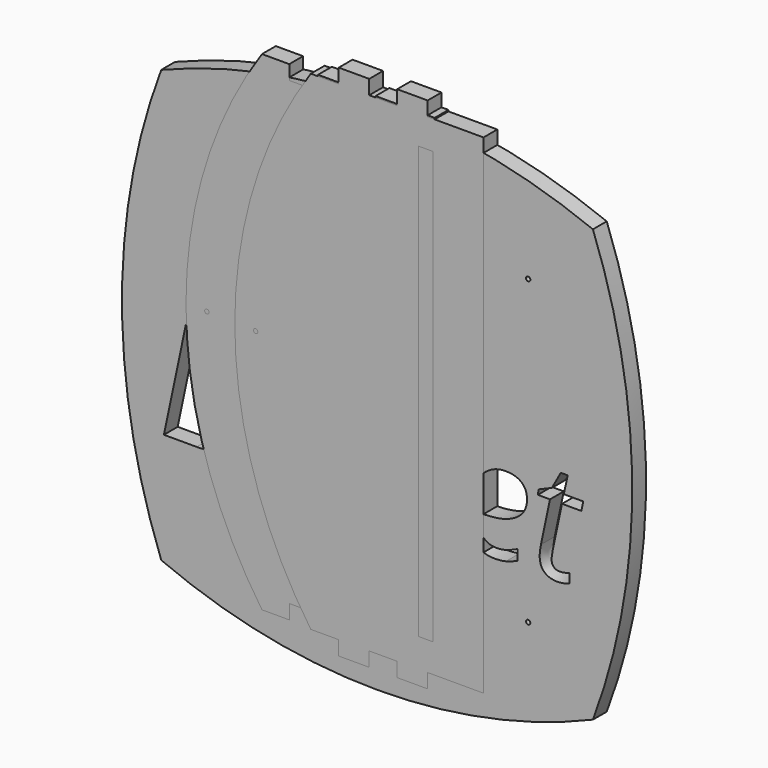
from build123d import *

# Parameters (mm, degrees)
F0_W     = 150
F0_H     = 150.000000298
F0_R     = 0.75
F3_DEPTH = 6
F1_R     = 0.75
F1_W     = 5
F1_H     = 150
F4_DEPTH = 6
F2_R     = 0.75
F2_W     = 5
F2_H     = 150
F5_DEPTH = 6


# Not quite as in the source:
# - ends of sketch curves that miss each other by under 0.0002 mm in the source are joined


with BuildPart() as f3:
    # F0 (on Front) → F3 (new body)
    with BuildSketch(Plane.XZ):
        with Locations((0, 1.49e-07)):
            Rectangle(F0_W, F0_H)
        with Locations((-52.5, -52.5)):
            Circle(F0_R, mode=Mode.SUBTRACT)
        with BuildLine():
            Line((-66.4784138573, -0.3075545752), (-57.236004571, -0.3075545752))
            add(Edge.make_bspline(
                [(-57.236004571, -0.3075545752), (-46.5898846592, -0.3075545752), (-46.5898846592, -8.5878700622)],
                knots=[0, 0, 0, 1, 1, 1], degree=2))
            add(Edge.make_bspline(
                [(-46.5898846592, -8.5878700622), (-46.5898846592, -12.0656025667), (-48.7309376637, -14.4550650358)],
                knots=[0, 0, 0, 1, 1, 1], degree=2))
            add(Edge.make_bspline(
                [(-48.7309376637, -14.4550650358), (-50.8719906682, -16.8445275048), (-54.7676819544, -17.562154847)],
                knots=[0, 0, 0, 1, 1, 1], degree=2))
            Line((-54.7676819544, -17.562154847), (-54.7676819544, -17.8066213043))
            add(Edge.make_bspline(
                [(-54.7676819544, -17.8066213043), (-51.9366026593, -18.5952227792), (-50.4185448201, -20.5312394002)],
                knots=[0, 0, 0, 1, 1, 1], degree=2))
            add(Edge.make_bspline(
                [(-50.4185448201, -20.5312394002), (-48.9004869808, -22.4672560212), (-48.9004869808, -25.1721590803)],
                knots=[0, 0, 0, 1, 1, 1], degree=2))
            add(Edge.make_bspline(
                [(-48.9004869808, -25.1721590803), (-48.9004869808, -30.4005868592), (-52.6463439868, -33.3696714123)],
                knots=[0, 0, 0, 1, 1, 1], degree=2))
            add(Edge.make_bspline(
                [(-52.6463439868, -33.3696714123), (-56.3922009928, -36.3387559655), (-62.6773547481, -36.3387559655)],
                knots=[0, 0, 0, 1, 1, 1], degree=2))
            Line((-62.6773547481, -36.3387559655), (-74.0884180906, -36.3387559655))
            Line((-74.0884180906, -36.3387559655), (-66.4784138573, -0.3075545752))
        make_face(mode=Mode.SUBTRACT)
        with BuildLine():
            add(Edge.make_bspline(
                [(-37.0280917755, -11.3243171802), (-33.9486030158, -8.8323365194), (-30.2737201426, -8.8323365194)],
                knots=[0, 0, 0, 1, 1, 1], degree=2))
            add(Edge.make_bspline(
                [(-30.2737201426, -8.8323365194), (-28.0104339095, -8.8323365194), (-26.2360805909, -10.0546688056)],
                knots=[0, 0, 0, 1, 1, 1], degree=2))
            add(Edge.make_bspline(
                [(-26.2360805909, -10.0546688056), (-24.4617272722, -11.2770010917), (-23.4759754285, -13.5639453691)],
                knots=[0, 0, 0, 1, 1, 1], degree=2))
            Line((-23.4759754285, -13.5639453691), (-23.1999649123, -13.5639453691))
            Line((-23.1999649123, -13.5639453691), (-21.5517878297, -9.3291554486))
            Line((-21.5517878297, -9.3291554486), (-18.4210399741, -9.3291554486))
            Line((-18.4210399741, -9.3291554486), (-24.1620587117, -36.3387559655))
            Line((-24.1620587117, -36.3387559655), (-27.4426408475, -36.3387559655))
            Line((-27.4426408475, -36.3387559655), (-26.7959876381, -31.1891883341))
            Line((-26.7959876381, -31.1891883341), (-26.9931380068, -31.1891883341))
            add(Edge.make_bspline(
                [(-26.9931380068, -31.1891883341), (-31.4093062665, -36.8355748947), (-36.2907493964, -36.8355748947)],
                knots=[0, 0, 0, 1, 1, 1], degree=2))
            add(Edge.make_bspline(
                [(-36.2907493964, -36.8355748947), (-39.7132797977, -36.8355748947), (-41.6611254408, -34.3948533298)],
                knots=[0, 0, 0, 1, 1, 1], degree=2))
            add(Edge.make_bspline(
                [(-41.6611254408, -34.3948533298), (-43.6089710839, -31.9541317648), (-43.6089710839, -27.7114558296)],
                knots=[0, 0, 0, 1, 1, 1], degree=2))
            add(Edge.make_bspline(
                [(-43.6089710839, -27.7114558296), (-43.6089710839, -22.5855462424), (-41.8582758095, -18.2009220417)],
                knots=[0, 0, 0, 1, 1, 1], degree=2))
            add(Edge.make_bspline(
                [(-41.8582758095, -18.2009220417), (-40.1075805352, -13.8162978411), (-37.0280917755, -11.3243171802)],
                knots=[0, 0, 0, 1, 1, 1], degree=2))
        make_face(mode=Mode.SUBTRACT)
        with BuildLine():
            add(Edge.make_bspline(
                [(0.0401205543, -25.9252734888), (0.6079136163, -27.1436627676), (0.6079136163, -28.673549629)],
                knots=[0, 0, 0, 1, 1, 1], degree=2))
            add(Edge.make_bspline(
                [(0.6079136163, -28.673549629), (0.6079136163, -32.5219248268), (-2.1167044796, -34.6787498607)],
                knots=[0, 0, 0, 1, 1, 1], degree=2))
            add(Edge.make_bspline(
                [(-2.1167044796, -34.6787498607), (-4.8413225756, -36.8355748947), (-9.7937398382, -36.8355748947)],
                knots=[0, 0, 0, 1, 1, 1], degree=2))
            add(Edge.make_bspline(
                [(-9.7937398382, -36.8355748947), (-13.9575556259, -36.8355748947), (-17.3091118945, -35.1321957088)],
                knots=[0, 0, 0, 1, 1, 1], degree=2))
            Line((-17.3091118945, -35.1321957088), (-17.3091118945, -31.2365044226))
            add(Edge.make_bspline(
                [(-17.3091118945, -31.2365044226), (-15.5820746643, -32.2695723548), (-13.5869129327, -32.8373654167)],
                knots=[0, 0, 0, 1, 1, 1], degree=2))
            add(Edge.make_bspline(
                [(-13.5869129327, -32.8373654167), (-11.5917512011, -33.4051584787), (-9.8883720152, -33.4051584787)],
                knots=[0, 0, 0, 1, 1, 1], degree=2))
            add(Edge.make_bspline(
                [(-9.8883720152, -33.4051584787), (-6.7891682187, -33.4051584787), (-5.2119652688, -32.1749401778)],
                knots=[0, 0, 0, 1, 1, 1], degree=2))
            add(Edge.make_bspline(
                [(-5.2119652688, -32.1749401778), (-3.6347623189, -30.9447218769), (-3.6347623189, -29.020534278)],
                knots=[0, 0, 0, 1, 1, 1], degree=2))
            add(Edge.make_bspline(
                [(-3.6347623189, -29.020534278), (-3.6347623189, -27.6168236526), (-4.4943379266, -26.6547298532)],
                knots=[0, 0, 0, 1, 1, 1], degree=2))
            add(Edge.make_bspline(
                [(-4.4943379266, -26.6547298532), (-5.3539135343, -25.6926360537), (-8.2165368883, -24.0129149121)],
                knots=[0, 0, 0, 1, 1, 1], degree=2))
            add(Edge.make_bspline(
                [(-8.2165368883, -24.0129149121), (-11.4182588766, -22.2149035492), (-12.7509953693, -20.4918093265)],
                knots=[0, 0, 0, 1, 1, 1], degree=2))
            add(Edge.make_bspline(
                [(-12.7509953693, -20.4918093265), (-14.0837318619, -18.7687151037), (-14.0837318619, -16.4029106789)],
                knots=[0, 0, 0, 1, 1, 1], degree=2))
            add(Edge.make_bspline(
                [(-14.0837318619, -16.4029106789), (-14.0837318619, -13.0040383219), (-11.5917512011, -10.9181874206)],
                knots=[0, 0, 0, 1, 1, 1], degree=2))
            add(Edge.make_bspline(
                [(-11.5917512011, -10.9181874206), (-9.0997705403, -8.8323365194), (-5.0384729443, -8.8323365194)],
                knots=[0, 0, 0, 1, 1, 1], degree=2))
            add(Edge.make_bspline(
                [(-5.0384729443, -8.8323365194), (-0.8194550534, -8.8323365194), (3.0998942771, -10.6618919413)],
                knots=[0, 0, 0, 1, 1, 1], degree=2))
            Line((3.0998942771, -10.6618919413), (1.7671577845, -14.037106254))
            Line((1.7671577845, -14.037106254), (0.3871052033, -13.4219971036))
            add(Edge.make_bspline(
                [(0.3871052033, -13.4219971036), (-2.1048754575, -12.3573851124), (-5.0384729443, -12.3573851124)],
                knots=[0, 0, 0, 1, 1, 1], degree=2))
            add(Edge.make_bspline(
                [(-5.0384729443, -12.3573851124), (-7.3254172217, -12.3573851124), (-8.6344956701, -13.4298831183)],
                knots=[0, 0, 0, 1, 1, 1], degree=2))
            add(Edge.make_bspline(
                [(-8.6344956701, -13.4298831183), (-9.9435741185, -14.5023811243), (-9.9435741185, -16.2057603101)],
                knots=[0, 0, 0, 1, 1, 1], degree=2))
            add(Edge.make_bspline(
                [(-9.9435741185, -16.2057603101), (-9.9435741185, -17.5858128913), (-9.0682264813, -18.571564735)],
                knots=[0, 0, 0, 1, 1, 1], degree=2))
            add(Edge.make_bspline(
                [(-9.0682264813, -18.571564735), (-8.1928788441, -19.5573165787), (-5.456431726, -21.1108614843)],
                knots=[0, 0, 0, 1, 1, 1], degree=2))
            add(Edge.make_bspline(
                [(-5.456431726, -21.1108614843), (-2.814616785, -22.5855462424), (-1.6711446463, -23.6462152262)],
                knots=[0, 0, 0, 1, 1, 1], degree=2))
            add(Edge.make_bspline(
                [(-1.6711446463, -23.6462152262), (-0.5276725076, -24.7068842101), (0.0401205543, -25.9252734888)],
                knots=[0, 0, 0, 1, 1, 1], degree=2))
        make_face(mode=Mode.SUBTRACT)
        with Locations((52.5, -52.5)):
            Circle(F0_R, mode=Mode.SUBTRACT)
        with BuildLine():
            Line((12.1451531948, -22.5618881982), (12.2397853718, -22.5618881982))
            Line((12.2397853718, -22.5618881982), (25.2043936199, -9.3291554486))
            Line((25.2043936199, -9.3291554486), (30.1568108825, -9.3291554486))
            Line((30.1568108825, -9.3291554486), (18.6037992746, -20.8348509681))
            Line((18.6037992746, -20.8348509681), (25.8668188588, -36.3387559655))
            Line((25.8668188588, -36.3387559655), (21.2613862451, -36.3387559655))
            Line((21.2613862451, -36.3387559655), (15.473051419, -23.4214638059))
            Line((15.473051419, -23.4214638059), (11.727194413, -26.4575794844))
            Line((11.727194413, -26.4575794844), (9.7004886224, -36.3387559655))
            Line((9.7004886224, -36.3387559655), (5.5130147905, -36.3387559655))
            Line((5.5130147905, -36.3387559655), (13.6434959972, 2.0109337611))
            Line((13.6434959972, 2.0109337611), (17.8388558439, 2.0109337611))
            add(Edge.make_bspline(
                [(17.8388558439, 2.0109337611), (16.0645025252, -6.2693817258), (14.6568488925, -12.82660299)],
                knots=[0, 0, 0, 1, 1, 1], degree=2))
            add(Edge.make_bspline(
                [(14.6568488925, -12.82660299), (13.2491952597, -19.3838242542), (12.1451531948, -22.5618881982)],
                knots=[0, 0, 0, 1, 1, 1], degree=2))
        make_face(mode=Mode.SUBTRACT)
        with BuildLine():
            add(Edge.make_bspline(
                [(44.7695962133, -36.4018440835), (42.9952428946, -36.8355748947), (40.8581328975, -36.8355748947)],
                knots=[0, 0, 0, 1, 1, 1], degree=2))
            add(Edge.make_bspline(
                [(40.8581328975, -36.8355748947), (36.3236744166, -36.8355748947), (33.7331185714, -34.1464438652)],
                knots=[0, 0, 0, 1, 1, 1], degree=2))
            add(Edge.make_bspline(
                [(33.7331185714, -34.1464438652), (31.1425627262, -31.4573128356), (31.1425627262, -26.7020459417)],
                knots=[0, 0, 0, 1, 1, 1], degree=2))
            add(Edge.make_bspline(
                [(31.1425627262, -26.7020459417), (31.1425627262, -22.0729552837), (32.9800041628, -17.8184503264)],
                knots=[0, 0, 0, 1, 1, 1], degree=2))
            add(Edge.make_bspline(
                [(32.9800041628, -17.8184503264), (34.8174455994, -13.5639453691), (37.8496182706, -11.1981409442)],
                knots=[0, 0, 0, 1, 1, 1], degree=2))
            add(Edge.make_bspline(
                [(37.8496182706, -11.1981409442), (40.8817909418, -8.8323365194), (44.525129756, -8.8323365194)],
                knots=[0, 0, 0, 1, 1, 1], degree=2))
            add(Edge.make_bspline(
                [(44.525129756, -8.8323365194), (48.2946448063, -8.8323365194), (50.1951743609, -10.4726275873)],
                knots=[0, 0, 0, 1, 1, 1], degree=2))
            add(Edge.make_bspline(
                [(50.1951743609, -10.4726275873), (52.0957039155, -12.1129186552), (52.0957039155, -15.046516142)],
                knots=[0, 0, 0, 1, 1, 1], degree=2))
            add(Edge.make_bspline(
                [(52.0957039155, -15.046516142), (52.0957039155, -19.4784564312), (48.0028622605, -22.0059241584)],
                knots=[0, 0, 0, 1, 1, 1], degree=2))
            add(Edge.make_bspline(
                [(48.0028622605, -22.0059241584), (43.9100206056, -24.5333918856), (36.2921303576, -24.5333918856)],
                knots=[0, 0, 0, 1, 1, 1], degree=2))
            Line((36.2921303576, -24.5333918856), (35.4798708384, -24.5333918856))
            Line((35.4798708384, -24.5333918856), (35.3852386614, -26.5048955729))
            add(Edge.make_bspline(
                [(35.3852386614, -26.5048955729), (35.3852386614, -29.7302756055), (36.8993534933, -31.5440589978)],
                knots=[0, 0, 0, 1, 1, 1], degree=2))
            add(Edge.make_bspline(
                [(36.8993534933, -31.5440589978), (38.4134683252, -33.3578423902), (41.5915322692, -33.3578423902)],
                knots=[0, 0, 0, 1, 1, 1], degree=2))
            add(Edge.make_bspline(
                [(41.5915322692, -33.3578423902), (43.1450771749, -33.3578423902), (44.7853682428, -32.9122825569)],
                knots=[0, 0, 0, 1, 1, 1], degree=2))
            add(Edge.make_bspline(
                [(44.7853682428, -32.9122825569), (46.4256593107, -32.4667227235), (48.8624378682, -31.2838205111)],
                knots=[0, 0, 0, 1, 1, 1], degree=2))
            Line((48.8624378682, -31.2838205111), (48.8624378682, -34.8877292516))
            add(Edge.make_bspline(
                [(48.8624378682, -34.8877292516), (46.5439495319, -35.9681132723), (44.7695962133, -36.4018440835)],
                knots=[0, 0, 0, 1, 1, 1], degree=2))
        make_face(mode=Mode.SUBTRACT)
        with BuildLine():
            add(Edge.make_bspline(
                [(61.3578282387, -32.7151321881), (62.0715125736, -33.4524745672), (63.349046963, -33.4524745672)],
                knots=[0, 0, 0, 1, 1, 1], degree=2))
            add(Edge.make_bspline(
                [(63.349046963, -33.4524745672), (64.7054414999, -33.4524745672), (66.8977536002, -32.8137073725)],
                knots=[0, 0, 0, 1, 1, 1], degree=2))
            Line((66.8977536002, -32.8137073725), (66.8977536002, -35.9917713165))
            add(Edge.make_bspline(
                [(66.8977536002, -35.9917713165), (66.0618360368, -36.3387559655), (64.8316177359, -36.5871654301)],
                knots=[0, 0, 0, 1, 1, 1], degree=2))
            add(Edge.make_bspline(
                [(64.8316177359, -36.5871654301), (63.601399435, -36.8355748947), (62.8601140485, -36.8355748947)],
                knots=[0, 0, 0, 1, 1, 1], degree=2))
            add(Edge.make_bspline(
                [(62.8601140485, -36.8355748947), (59.7766822815, -36.8355748947), (58.140334221, -35.3687761513)],
                knots=[0, 0, 0, 1, 1, 1], degree=2))
            add(Edge.make_bspline(
                [(58.140334221, -35.3687761513), (56.5039861605, -33.9019774079), (56.5039861605, -30.9920379654)],
                knots=[0, 0, 0, 1, 1, 1], degree=2))
            add(Edge.make_bspline(
                [(56.5039861605, -30.9920379654), (56.5039861605, -29.367518927), (56.9456029864, -27.2934970479)],
                knots=[0, 0, 0, 1, 1, 1], degree=2))
            Line((56.9456029864, -27.2934970479), (60.076350842, -12.4599033041))
            Line((60.076350842, -12.4599033041), (55.8336749068, -12.4599033041))
            Line((55.8336749068, -12.4599033041), (56.1806595557, -10.6618919413))
            Line((56.1806595557, -10.6618919413), (60.7387760809, -8.7377043424))
            Line((60.7387760809, -8.7377043424), (63.822207848, -3.114975826))
            Line((63.822207848, -3.114975826), (66.2353283613, -3.114975826))
            Line((66.2353283613, -3.114975826), (64.8789338244, -9.3291554486))
            Line((64.8789338244, -9.3291554486), (71.6293624499, -9.3291554486))
            Line((71.6293624499, -9.3291554486), (70.9905952552, -12.4599033041))
            Line((70.9905952552, -12.4599033041), (64.2638246739, -12.4599033041))
            Line((64.2638246739, -12.4599033041), (61.0857607299, -27.3408131364))
            add(Edge.make_bspline(
                [(61.0857607299, -27.3408131364), (60.6441439039, -29.4858091482), (60.6441439039, -30.5977372279)],
                knots=[0, 0, 0, 1, 1, 1], degree=2))
            add(Edge.make_bspline(
                [(60.6441439039, -30.5977372279), (60.6441439039, -31.9777898091), (61.3578282387, -32.7151321881)],
                knots=[0, 0, 0, 1, 1, 1], degree=2))
        make_face(mode=Mode.SUBTRACT)
        Polygon((-9.8206784108, 13.3505715057), (-23.3275989091, 13.3505715057), (-17.6531634364, 40.217406402), (-14.5248736214, 40.217406402), (-19.5995242048, 16.1789688761), (-9.2150132775, 16.1789688761), align=None, mode=Mode.SUBTRACT)
        Polygon((1.4047074104, 33.4904072509), (-2.8996312073, 13.3505715057), (-5.9867593142, 13.3505715057), (-1.6824206965, 33.4904072509), align=None, mode=Mode.SUBTRACT)
        with Locations((-52.5, 52.5)):
            Circle(F0_R, mode=Mode.SUBTRACT)
        with BuildLine():
            add(Edge.make_bspline(
                [(4.4918355173, 5.906182585), (3.004133782, 4.3067562134), (0.5755930045, 4.3067562134)],
                knots=[0, 0, 0, 1, 1, 1], degree=2))
            add(Edge.make_bspline(
                [(0.5755930045, 4.3067562134), (-0.6945397023, 4.3067562134), (-1.7235824046, 4.6948523183)],
                knots=[0, 0, 0, 1, 1, 1], degree=2))
            Line((-1.7235824046, 4.6948523183), (-1.7235824046, 7.2880399281))
            add(Edge.make_bspline(
                [(-1.7235824046, 7.2880399281), (-0.547533602, 6.8823030912), (0.334503, 6.8823030912)],
                knots=[0, 0, 0, 1, 1, 1], degree=2))
            add(Edge.make_bspline(
                [(0.334503, 6.8823030912), (1.7340010751, 6.8823030912), (2.4866723088, 8.0201303078)],
                knots=[0, 0, 0, 1, 1, 1], degree=2))
            add(Edge.make_bspline(
                [(2.4866723088, 8.0201303078), (3.2393435425, 9.1579575243), (3.6980025755, 11.2748453691)],
                knots=[0, 0, 0, 1, 1, 1], degree=2))
            Line((3.6980025755, 11.2748453691), (7.8729758249, 31.1559503777))
            Line((7.8729758249, 31.1559503777), (4.3271886849, 31.1559503777))
            Line((4.3271886849, 31.1559503777), (4.5623984455, 32.3908016204))
            Line((4.5623984455, 32.3908016204), (8.34927559, 33.6021318872))
            Line((8.34927559, 33.6021318872), (8.7726531589, 35.4367680193))
            add(Edge.make_bspline(
                [(8.7726531589, 35.4367680193), (9.6194082968, 39.1119205275), (11.1159303982, 40.6290234829)],
                knots=[0, 0, 0, 1, 1, 1], degree=2))
            add(Edge.make_bspline(
                [(11.1159303982, 40.6290234829), (12.6124524995, 42.1461264383), (15.5525745061, 42.1461264383)],
                knots=[0, 0, 0, 1, 1, 1], degree=2))
            add(Edge.make_bspline(
                [(15.5525745061, 42.1461264383), (16.2876050078, 42.1461264383), (17.3519291742, 41.9344376539)],
                knots=[0, 0, 0, 1, 1, 1], degree=2))
            add(Edge.make_bspline(
                [(17.3519291742, 41.9344376539), (18.4162533405, 41.7227488694), (19.0042777419, 41.4640181328)],
                knots=[0, 0, 0, 1, 1, 1], degree=2))
            Line((19.0042777419, 41.4640181328), (18.2163250441, 39.0942797955))
            add(Edge.make_bspline(
                [(18.2163250441, 39.0942797955), (16.822707213, 39.6293820007), (15.6995806065, 39.6293820007)],
                knots=[0, 0, 0, 1, 1, 1], degree=2))
            add(Edge.make_bspline(
                [(15.6995806065, 39.6293820007), (14.1001542349, 39.6293820007), (13.2445787309, 38.7385250327)],
                knots=[0, 0, 0, 1, 1, 1], degree=2))
            add(Edge.make_bspline(
                [(13.2445787309, 38.7385250327), (12.389003227, 37.8476680647), (11.8597812658, 35.4779297274)],
                knots=[0, 0, 0, 1, 1, 1], degree=2))
            Line((11.8597812658, 35.4779297274), (11.4011222328, 33.4904072509))
            Line((11.4011222328, 33.4904072509), (15.7701435346, 33.4904072509))
            Line((15.7701435346, 33.4904072509), (15.3114845016, 31.1559503777))
            Line((15.3114845016, 31.1559503777), (10.9601039318, 31.1559503777))
            Line((10.9601039318, 31.1559503777), (6.6969270223, 10.9808331684))
            add(Edge.make_bspline(
                [(6.6969270223, 10.9808331684), (5.9795372526, 7.5056089566), (4.4918355173, 5.906182585)],
                knots=[0, 0, 0, 1, 1, 1], degree=2))
        make_face(mode=Mode.SUBTRACT)
        with BuildLine():
            add(Edge.make_bspline(
                [(20.0362605662, 16.0525436298), (20.5684226494, 15.5027408146), (21.5210221795, 15.5027408146)],
                knots=[0, 0, 0, 1, 1, 1], degree=2))
            add(Edge.make_bspline(
                [(21.5210221795, 15.5027408146), (22.5324241498, 15.5027408146), (24.1671319855, 15.9790405796)],
                knots=[0, 0, 0, 1, 1, 1], degree=2))
            Line((24.1671319855, 15.9790405796), (24.1671319855, 13.6093022423))
            add(Edge.make_bspline(
                [(24.1671319855, 13.6093022423), (23.5438261201, 13.3505715057), (22.626508054, 13.1653438193)],
                knots=[0, 0, 0, 1, 1, 1], degree=2))
            add(Edge.make_bspline(
                [(22.626508054, 13.1653438193), (21.7091899879, 12.9801161329), (21.1564470507, 12.9801161329)],
                knots=[0, 0, 0, 1, 1, 1], degree=2))
            add(Edge.make_bspline(
                [(21.1564470507, 12.9801161329), (18.8572716415, 12.9801161329), (17.6371210088, 14.0738415193)],
                knots=[0, 0, 0, 1, 1, 1], degree=2))
            add(Edge.make_bspline(
                [(17.6371210088, 14.0738415193), (16.4169703761, 15.1675669058), (16.4169703761, 17.3373769467)],
                knots=[0, 0, 0, 1, 1, 1], degree=2))
            add(Edge.make_bspline(
                [(16.4169703761, 17.3373769467), (16.4169703761, 18.5487072134), (16.7462640408, 20.0952113889)],
                knots=[0, 0, 0, 1, 1, 1], degree=2))
            Line((16.7462640408, 20.0952113889), (19.080720914, 31.1559503777))
            Line((19.080720914, 31.1559503777), (15.9171496349, 31.1559503777))
            Line((15.9171496349, 31.1559503777), (16.1758803715, 32.4966460127))
            Line((16.1758803715, 32.4966460127), (19.5746614111, 33.9314255519))
            Line((19.5746614111, 33.9314255519), (21.8738368203, 38.1240395333))
            Line((21.8738368203, 38.1240395333), (23.6731914883, 38.1240395333))
            Line((23.6731914883, 38.1240395333), (22.6617895181, 33.4904072509))
            Line((22.6617895181, 33.4904072509), (27.6952783934, 33.4904072509))
            Line((27.6952783934, 33.4904072509), (27.2189786283, 31.1559503777))
            Line((27.2189786283, 31.1559503777), (22.203130485, 31.1559503777))
            Line((22.203130485, 31.1559503777), (19.8333921477, 20.0599299248))
            add(Edge.make_bspline(
                [(19.8333921477, 20.0599299248), (19.504098483, 18.4605035532), (19.504098483, 17.6313891473)],
                knots=[0, 0, 0, 1, 1, 1], degree=2))
            add(Edge.make_bspline(
                [(19.504098483, 17.6313891473), (19.504098483, 16.602346445), (20.0362605662, 16.0525436298)],
                knots=[0, 0, 0, 1, 1, 1], degree=2))
        make_face(mode=Mode.SUBTRACT)
        with BuildLine():
            add(Edge.make_bspline(
                [(-0.3417250615, 37.3566676896), (-0.8180248266, 37.8065063566), (-0.8180248266, 38.6356207625)],
                knots=[0, 0, 0, 1, 1, 1], degree=2))
            add(Edge.make_bspline(
                [(-0.8180248266, 38.6356207625), (-0.8180248266, 39.6646634648), (-0.2300004253, 40.3173705502)],
                knots=[0, 0, 0, 1, 1, 1], degree=2))
            add(Edge.make_bspline(
                [(-0.2300004253, 40.3173705502), (0.358023976, 40.9700776357), (1.2929827741, 40.9700776357)],
                knots=[0, 0, 0, 1, 1, 1], degree=2))
            add(Edge.make_bspline(
                [(1.2929827741, 40.9700776357), (2.9100498778, 40.9700776357), (2.9100498778, 39.317729068)],
                knots=[0, 0, 0, 1, 1, 1], degree=2))
            add(Edge.make_bspline(
                [(2.9100498778, 39.317729068), (2.9100498778, 38.3063270977), (2.2955643784, 37.6065780601)],
                knots=[0, 0, 0, 1, 1, 1], degree=2))
            add(Edge.make_bspline(
                [(2.2955643784, 37.6065780601), (1.681078879, 36.9068290226), (0.8696052052, 36.9068290226)],
                knots=[0, 0, 0, 1, 1, 1], degree=2))
            add(Edge.make_bspline(
                [(0.8696052052, 36.9068290226), (0.1345747035, 36.9068290226), (-0.3417250615, 37.3566676896)],
                knots=[0, 0, 0, 1, 1, 1], degree=2))
        make_face(mode=Mode.SUBTRACT)
        with Locations((52.5, 52.5)):
            Circle(F0_R, mode=Mode.SUBTRACT)
        with BuildLine():
            ThreePointArc((75, 75.000000298), (-2.88e-08, 89.4985285534), (-75, 75))
            Line((-75, 75), (75, 75.000000298))
        make_face()
        with BuildLine():
            Line((-75, -75), (-75, 75))
            ThreePointArc((-75, 75), (-88.6491712085, -3.0074e-06), (-75, -75))
        make_face()
        with BuildLine():
            Line((75, -75), (-75, -75))
            ThreePointArc((-75, -75), (0, -90.2725273781), (75, -75))
        make_face()
        with BuildLine():
            ThreePointArc((74.9999931729, -74.9999970198), (88.6491640834, 3.0074e-06), (74.9999928749, 75.0000029802))
            Line((74.9999928749, 75.0000029802), (74.9999931729, -74.9999970198))
        make_face()
    extrude(amount=F3_DEPTH)


with BuildPart() as f4:
    # F1 (on Front) → F4 (new body)
    with BuildSketch(Plane.XZ):
        with BuildLine():
            Line((20.0000001626, -78.7899424732), (19.9999998374, 91.2100575268))
            Line((19.9999998374, 91.2100575268), (-0.5218474052, 91.2100575268))
            Line((-0.5218474052, 91.2100575268), (-0.5218474052, 88.210016489))
            Line((-0.5218474052, 88.210016489), (-0.5218474052, 86.2100575268))
            Line((-0.5218474052, 86.2100575268), (-10.5218474052, 86.2100575268))
            Line((-10.5218474052, 86.2100575268), (-10.5218474052, 88.210016489))
            Line((-10.5218474052, 88.210016489), (-10.5218474052, 91.2100575268))
            Line((-10.5218474052, 91.2100575268), (-20.5218474052, 91.2100575268))
            Line((-20.5218474052, 91.2100575268), (-20.5218474052, 88.210016489))
            Line((-20.5218474052, 88.210016489), (-20.5218474052, 86.2100575268))
            Line((-20.5218474052, 86.2100575268), (-30.5218474052, 86.2100575268))
            Line((-30.5218474052, 86.2100575268), (-30.5218474052, 88.210016489))
            Line((-30.5218474052, 88.210016489), (-30.5218474052, 91.2100575268))
            Line((-30.5218474052, 91.2100575268), (-40.0000001626, 91.2100575268))
            ThreePointArc((-40.0000001626, 91.2100575268), (-66.4079290569, 6.2100574763), (-39.9999998374, -78.7899424732))
            Line((-39.9999998374, -78.7899424732), (-30.5218463486, -78.7899435368))
            Line((-30.5218463486, -78.7899435368), (-30.5218463486, -75.7881775498))
            Line((-30.5218463486, -75.7881775498), (-30.5218463486, -73.7881775498))
            Line((-30.5218463486, -73.7881775498), (-20.5218463486, -73.7881775498))
            Line((-20.5218463486, -73.7881775498), (-20.5218463486, -75.7881775498))
            Line((-20.5218463486, -75.7881775498), (-20.5218463486, -78.7899435368))
            Line((-20.5218463486, -78.7899435368), (-10.5218463486, -78.7899435368))
            Line((-10.5218463486, -78.7899435368), (-10.5218463486, -75.7881775498))
            Line((-10.5218463486, -75.7881775498), (-10.5218463486, -73.7881775498))
            Line((-10.5218463486, -73.7881775498), (-0.5218463486, -73.7881775498))
            Line((-0.5218463486, -73.7881775498), (-0.5218463486, -75.7881775498))
            Line((-0.5218463486, -75.7881775498), (-0.5218463486, -78.7899435368))
            Line((-0.5218463486, -78.7899435368), (20.0000001626, -78.7899424732))
        make_face()
        with Locations((-59.1692306225, 6.2100575268)):
            Circle(F1_R, mode=Mode.SUBTRACT)
        with Locations((0, 6.2100574885)):
            Rectangle(F1_W, F1_H, mode=Mode.SUBTRACT)
    extrude(amount=F4_DEPTH)


with BuildPart() as f5:
    # F2 (on Front) → F5 (new body)
    with BuildSketch(Plane.XZ):
        with BuildLine():
            Line((36.9674778498, -79.2646374009), (36.9674775247, 90.7353625991))
            Line((36.9674775247, 90.7353625991), (17.5674764112, 90.73536098))
            Line((17.5674764112, 90.73536098), (17.5674764112, 93.7375798821))
            Line((17.5674764112, 93.7375798821), (17.5674764112, 95.7375798821))
            Line((17.5674764112, 95.7375798821), (6.9674764112, 95.7375798821))
            Line((6.9674764112, 95.7375798821), (6.9674764112, 93.7375798821))
            Line((6.9674764112, 93.7375798821), (6.9674764112, 90.73536098))
            Line((6.9674764112, 90.73536098), (-2.7325235888, 90.73536098))
            Line((-2.7325235888, 90.73536098), (-2.7325235888, 93.7375798821))
            Line((-2.7325235888, 93.7375798821), (-2.7325235888, 95.7375798821))
            Line((-2.7325235888, 95.7375798821), (-13.3325235888, 95.7375798821))
            Line((-13.3325235888, 95.7375798821), (-13.3325235888, 93.7375798821))
            Line((-13.3325235888, 93.7375798821), (-13.3325235888, 90.73536098))
            Line((-13.3325235888, 90.73536098), (-23.0325235888, 90.73536098))
            ThreePointArc((-23.0325235888, 90.73536098), (-49.4404513696, 5.7353625486), (-23.0325221502, -79.2646374009))
            Line((-23.0325221502, -79.2646374009), (-13.3325221502, -79.2646374009))
            Line((-13.3325221502, -79.2646374009), (-13.3325221502, -82.2646374009))
            Line((-13.3325221502, -82.2646374009), (-13.3325221502, -84.2646374009))
            Line((-13.3325221502, -84.2646374009), (-2.7325221502, -84.2646374009))
            Line((-2.7325221502, -84.2646374009), (-2.7325221502, -82.2646374009))
            Line((-2.7325221502, -82.2646374009), (-2.7325221502, -79.2646374009))
            Line((-2.7325221502, -79.2646374009), (6.9674778498, -79.2646374009))
            Line((6.9674778498, -79.2646374009), (6.9674778498, -82.2646374009))
            Line((6.9674778498, -82.2646374009), (6.9674778498, -84.2646374009))
            Line((6.9674778498, -84.2646374009), (17.5674778498, -84.2646374009))
            Line((17.5674778498, -84.2646374009), (17.5674778498, -82.2646374009))
            Line((17.5674778498, -82.2646374009), (17.5674778498, -79.2646374009))
            Line((17.5674778498, -79.2646374009), (36.9674778498, -79.2646374009))
        make_face()
        with Locations((-42.2017529352, 5.7353625991)):
            Circle(F2_R, mode=Mode.SUBTRACT)
        with Locations((16.9674776873, 5.7353625608)):
            Rectangle(F2_W, F2_H, mode=Mode.SUBTRACT)
    extrude(amount=F5_DEPTH)


solid = Compound([f3.part, f4.part, f5.part])
